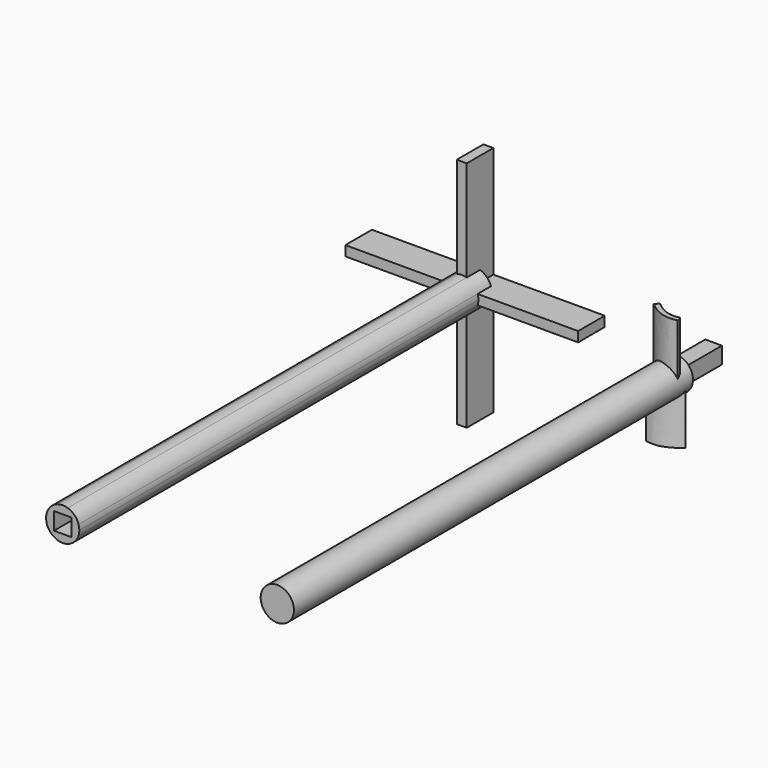
from build123d import *

# Parameters (mm, degrees)
F0_R      = 5
F0_W      = 5
F0_H      = 5
F1_DEPTH  = 150
F0_W_2    = 3
F0_H_2    = 3
F2_DEPTH  = 150
F3_DEPTH  = 10
F4_DEPTH  = 5
F5_DEPTH  = 14
F9_DEPTH  = 17.5
F10_DEPTH = 17.5
F11_W     = 5.2
F11_H     = 5.2
F12_DEPTH = 15


# Not quite as in the source:
# - ends of sketch curves that miss each other by under 0.0002 mm in the source are joined
# - the dataset's text gives a spline's control points without its knots; the knots are read off the source's solid
# - a feature names something its author has since deleted; it is built from what else it names


with BuildPart() as f1:
    # F0 (on Front) → F1 (new body)
    with BuildSketch(Plane.XZ):
        with Locations((64.5359467268, -0.1232206572)):
            Circle(F0_R)
        with Locations((64.5359467268, -0.1232206572)):
            Rectangle(F0_W, F0_H, mode=Mode.SUBTRACT)
        with Locations((64.5359467268, -0.1232206572)):
            Rectangle(F0_W, F0_H)
    extrude(amount=F1_DEPTH)

    # F0 (on Front) → F5 (join)
    with BuildSketch(Plane.XZ):
        with Locations((64.5359467268, -0.1232206572)):
            Rectangle(F0_W, F0_H)
    extrude(amount=-F5_DEPTH)

    # F7 (on Top) → F9 (join)
    with BuildSketch(Plane.XY):
        with BuildLine():
            Line((60.2211986423, -3.7655206016), (59.4354718924, -5.1162280142))
            add(Edge.make_bspline(
                [(59.4354718924, -5.1162280142), (61.0842581652, -5.5715008798), (64.452106893, -5.4157207464), (67.4619618477, -3.4758949633), (69.0351650119, -2.1422058344)],
                knots=[0, 0, 0, 0, 0.4813561613, 1, 1, 1, 1], degree=3))
            Line((69.0351650119, -2.1422058344), (67.9586756002, -1.0878058335))
            add(Edge.make_bspline(
                [(60.2211986423, -3.7655206016), (60.79518409, -3.8901325795), (62.0458350632, -3.9928459488), (63.6051513202, -3.6922198414), (64.9450123041, -3.1383545358), (66.2695568548, -2.4049913477), (67.2806730234, -1.6559071736), (67.9586756002, -1.0878058335)],
                knots=[0.0456486225, 0.0456486225, 0.0456486225, 0.0456486225, 0.25, 0.5, 0.625, 0.75, 0.9875741574, 0.9875741574, 0.9875741574, 0.9875741574], degree=3))
        make_face()
    extrude(amount=-F9_DEPTH)

    # F8 (on Top) → F10 (join)
    with BuildSketch(Plane.XY):
        with BuildLine():
            add(Edge.make_bspline(
                [(69.0762884915, -5.1635340787), (67.4275022186, -5.6188069444), (64.0596534908, -5.4630268109), (61.0497985361, -3.5232010278), (59.476595372, -2.1895118989)],
                knots=[0, 0, 0, 0, 0.4813561613, 1, 1, 1, 1], degree=3))
            Line((69.0762884915, -5.1635340787), (68.6770402906, -3.7176430476))
            add(Edge.make_bspline(
                [(68.6770402906, -3.7176430476), (67.9681620888, -3.913382796), (66.5887879598, -4.063839137), (64.9066090636, -3.7395259059), (63.5667480798, -3.1856606003), (62.2084474698, -2.4336076285), (61.1617523711, -1.6516299589), (60.4465751998, -1.0453357178)],
                knots=[0, 0, 0, 0, 0.25, 0.5, 0.625, 0.75, 1, 1, 1, 1], degree=3))
            Line((60.4465751998, -1.0453357178), (59.476595372, -2.1895118989))
        make_face()
    extrude(amount=F10_DEPTH)


with BuildPart() as f2:
    # F0 (on Front) → F2 (new body)
    with BuildSketch(Plane.XZ):
        with BuildLine():
            ThreePointArc((4.7696960071, -1.5), (4.9420886291, -0.7587884964), (5, 0))
            ThreePointArc((5, 0), (4.9420886291, 0.7587884964), (4.7696960071, 1.5))
            Line((4.7696960071, 1.5), (1.5, 1.5))
            Line((1.5, 1.5), (1.5, -1.5))
            Line((1.5, -1.5), (4.7696960071, -1.5))
        make_face()
        with BuildLine():
            Line((1.5, 1.5), (4.7696960071, 1.5))
            ThreePointArc((4.7696960071, 1.5), (3.5355339059, 3.5355339059), (1.5, 4.7696960071))
            Line((1.5, 4.7696960071), (1.5, 1.5))
        make_face()
        with BuildLine():
            Line((1.5, 1.5), (1.5, 4.7696960071))
            ThreePointArc((1.5, 4.7696960071), (0, 5), (-1.5, 4.7696960071))
            Line((-1.5, 4.7696960071), (-1.5, 1.5))
            Line((-1.5, 1.5), (1.5, 1.5))
        make_face()
        with BuildLine():
            Line((-1.5, 1.5), (-1.5, 4.7696960071))
            ThreePointArc((-1.5, 4.7696960071), (-3.5355339059, 3.5355339059), (-4.7696960071, 1.5))
            Line((-4.7696960071, 1.5), (-1.5, 1.5))
        make_face()
        with BuildLine():
            Line((-1.5, -1.5), (-1.5, 1.5))
            Line((-1.5, 1.5), (-4.7696960071, 1.5))
            ThreePointArc((-4.7696960071, 1.5), (-5, 0), (-4.7696960071, -1.5))
            Line((-4.7696960071, -1.5), (-1.5, -1.5))
        make_face()
        Rectangle(F0_W_2, F0_H_2)
        with BuildLine():
            ThreePointArc((1.5, -4.7696960071), (3.5355339059, -3.5355339059), (4.7696960071, -1.5))
            Line((4.7696960071, -1.5), (1.5, -1.5))
            Line((1.5, -1.5), (1.5, -4.7696960071))
        make_face()
        with BuildLine():
            ThreePointArc((-1.5, -4.7696960071), (0, -5), (1.5, -4.7696960071))
            Line((1.5, -4.7696960071), (1.5, -1.5))
            Line((1.5, -1.5), (-1.5, -1.5))
            Line((-1.5, -1.5), (-1.5, -4.7696960071))
        make_face()
        with BuildLine():
            ThreePointArc((-4.7696960071, -1.5), (-3.5355339059, -3.5355339059), (-1.5, -4.7696960071))
            Line((-1.5, -4.7696960071), (-1.5, -1.5))
            Line((-1.5, -1.5), (-4.7696960071, -1.5))
        make_face()
    extrude(amount=F2_DEPTH)

    # F0 (on Front) → F3 (join)
    with BuildSketch(Plane.XZ):
        with BuildLine():
            ThreePointArc((-4.7696960071, -1.5), (-5, 0), (-4.7696960071, 1.5))
            Line((-4.7696960071, 1.5), (-35, 1.5))
            Line((-35, 1.5), (-35, -1.5))
            Line((-35, -1.5), (-4.7696960071, -1.5))
        make_face()
        with BuildLine():
            ThreePointArc((-1.5, 4.7696960071), (0, 5), (1.5, 4.7696960071))
            Line((1.5, 4.7696960071), (1.5, 35))
            Line((1.5, 35), (-1.5, 35))
            Line((-1.5, 35), (-1.5, 4.7696960071))
        make_face()
        with BuildLine():
            Line((-1.5, -1.5), (-1.5, 1.5))
            Line((-1.5, 1.5), (-4.7696960071, 1.5))
            ThreePointArc((-4.7696960071, 1.5), (-5, 0), (-4.7696960071, -1.5))
            Line((-4.7696960071, -1.5), (-1.5, -1.5))
        make_face()
        with BuildLine():
            Line((1.5, 1.5), (1.5, 4.7696960071))
            ThreePointArc((1.5, 4.7696960071), (0, 5), (-1.5, 4.7696960071))
            Line((-1.5, 4.7696960071), (-1.5, 1.5))
            Line((-1.5, 1.5), (1.5, 1.5))
        make_face()
        Rectangle(F0_W_2, F0_H_2)
        with BuildLine():
            Line((1.5, -35), (1.5, -4.7696960071))
            ThreePointArc((1.5, -4.7696960071), (0, -5), (-1.5, -4.7696960071))
            Line((-1.5, -4.7696960071), (-1.5, -35))
            Line((-1.5, -35), (1.5, -35))
        make_face()
        with BuildLine():
            ThreePointArc((-1.5, -4.7696960071), (0, -5), (1.5, -4.7696960071))
            Line((1.5, -4.7696960071), (1.5, -1.5))
            Line((1.5, -1.5), (-1.5, -1.5))
            Line((-1.5, -1.5), (-1.5, -4.7696960071))
        make_face()
        with BuildLine():
            ThreePointArc((4.7696960071, -1.5), (4.9420886291, -0.7587884964), (5, 0))
            ThreePointArc((5, 0), (4.9420886291, 0.7587884964), (4.7696960071, 1.5))
            Line((4.7696960071, 1.5), (1.5, 1.5))
            Line((1.5, 1.5), (1.5, -1.5))
            Line((1.5, -1.5), (4.7696960071, -1.5))
        make_face()
        with BuildLine():
            ThreePointArc((4.7696960071, 1.5), (4.9420886291, 0.7587884964), (5, 0))
            ThreePointArc((5, 0), (4.9420886291, -0.7587884964), (4.7696960071, -1.5))
            Line((4.7696960071, -1.5), (35, -1.5))
            Line((35, -1.5), (35, 1.5))
            Line((35, 1.5), (4.7696960071, 1.5))
        make_face()
    extrude(amount=-F3_DEPTH)

    # F0 (on Front) → F4 (join)
    with BuildSketch(Plane.XZ):
        with BuildLine():
            Line((1.5, 1.5), (4.7696960071, 1.5))
            ThreePointArc((4.7696960071, 1.5), (3.5355339059, 3.5355339059), (1.5, 4.7696960071))
            Line((1.5, 4.7696960071), (1.5, 1.5))
        make_face()
        with BuildLine():
            ThreePointArc((1.5, -4.7696960071), (3.5355339059, -3.5355339059), (4.7696960071, -1.5))
            Line((4.7696960071, -1.5), (1.5, -1.5))
            Line((1.5, -1.5), (1.5, -4.7696960071))
        make_face()
        with BuildLine():
            Line((-1.5, 1.5), (-1.5, 4.7696960071))
            ThreePointArc((-1.5, 4.7696960071), (-3.5355339059, 3.5355339059), (-4.7696960071, 1.5))
            Line((-4.7696960071, 1.5), (-1.5, 1.5))
        make_face()
        with BuildLine():
            Line((-1.5, -1.5), (-1.5, 1.5))
            Line((-1.5, 1.5), (-4.7696960071, 1.5))
            ThreePointArc((-4.7696960071, 1.5), (-5, 0), (-4.7696960071, -1.5))
            Line((-4.7696960071, -1.5), (-1.5, -1.5))
        make_face()
        with BuildLine():
            ThreePointArc((-4.7696960071, -1.5), (-3.5355339059, -3.5355339059), (-1.5, -4.7696960071))
            Line((-1.5, -4.7696960071), (-1.5, -1.5))
            Line((-1.5, -1.5), (-4.7696960071, -1.5))
        make_face()
    extrude(amount=-F4_DEPTH)

    # F11 (on face) → F12 (cut)
    with BuildSketch(Plane.XZ.offset(150)):
        Rectangle(F11_W, F11_H)
    extrude(amount=-F12_DEPTH, mode=Mode.SUBTRACT)


solid = Compound([f1.part, f2.part])
